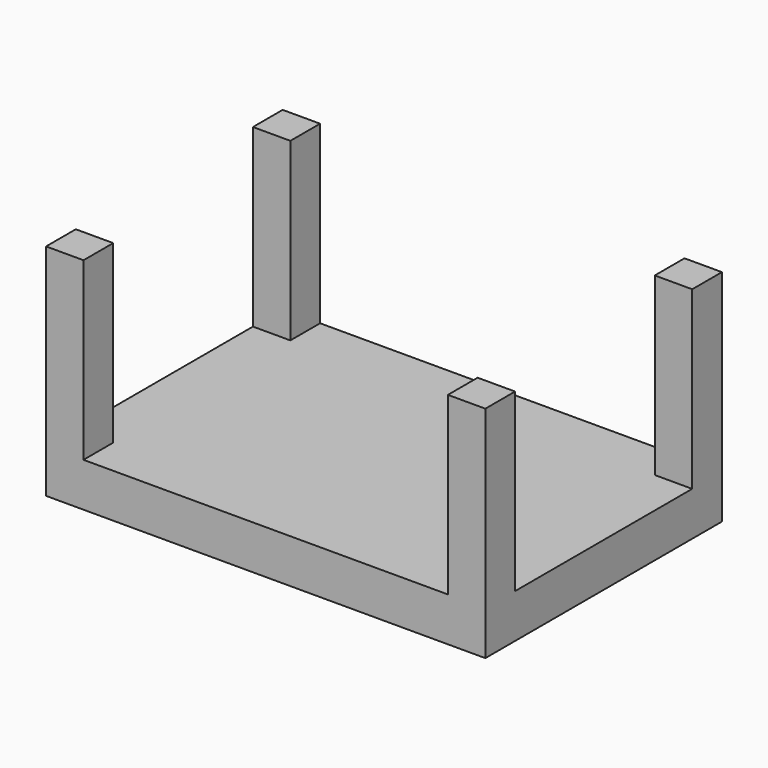
from build123d import *

# Parameters (mm, degrees)
F0_W     = 4.2595966585
F0_H     = 4.2287140257
F1_DEPTH = 5
F2_DEPTH = 25


with BuildPart() as f1:
    # F0 (on Top) → F1 (new body)
    with BuildSketch(Plane.XY):
        with Locations((-22.8702016707, 14.7173251896)):
            Rectangle(F0_W, F0_H)
        Polygon((20.7404033415, 16.8316822024), (-20.7404033415, 16.8316822024), (-20.7404033415, 12.6029681767), (-25, 12.6029681767), (-25, -12.6029681767), (-20.7404033415, -12.6029681767), (-20.7404033415, -16.8316822024), (20.7404033415, -16.8316822024), (20.7404033415, -12.6029681767), (25, -12.6029681767), (25, 12.6029681767), (20.7404033415, 12.6029681767), align=None)
        with Locations((22.8702016707, 14.7173251896)):
            Rectangle(F0_W, F0_H)
        with Locations((-22.8702016707, -14.7173251896)):
            Rectangle(F0_W, F0_H)
        with Locations((22.8702016707, -14.7173251896)):
            Rectangle(F0_W, F0_H)
    extrude(amount=F1_DEPTH)

    # F0 (on Top) → F2 (join)
    with BuildSketch(Plane.XY):
        with Locations((22.8702016707, 14.7173251896)):
            Rectangle(F0_W, F0_H)
        with Locations((22.8702016707, -14.7173251896)):
            Rectangle(F0_W, F0_H)
        with Locations((-22.8702016707, -14.7173251896)):
            Rectangle(F0_W, F0_H)
        with Locations((-22.8702016707, 14.7173251896)):
            Rectangle(F0_W, F0_H)
    extrude(amount=F2_DEPTH)


solid = f1.part
